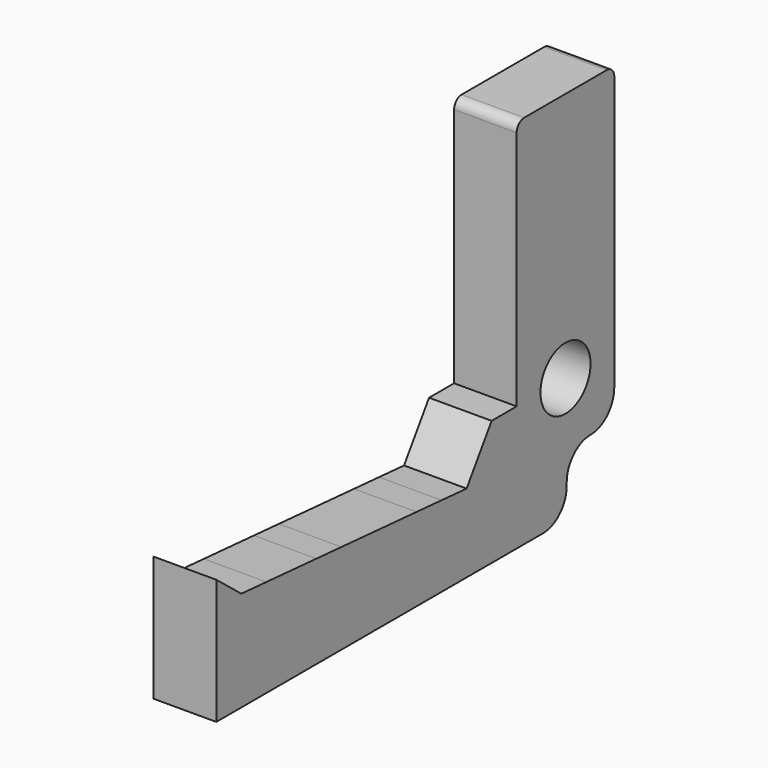
from build123d import *

# Parameters (mm, degrees)
F0_W      = 5.08
F0_H      = 9.906
F1_DEPTH  = 25.4
F2_W      = 5.08
F2_H      = 5.08
F3_DEPTH  = 5.08
F4_W      = 5.08
F4_H      = 5.08
F5_DEPTH  = 5.08
F6_DEPTH  = 5.08
F7_DEPTH  = 25.4
F9_DEPTH  = 5.081
F10_R     = 2.41299
F11_R     = 2.54
F12_DEPTH = 5.081
F13_R     = 0.762


# Not quite as in the source:
# - a fillet or chamfer is up to 0.001 mm smaller than in the source, because OpenCascade refuses the exact size


with BuildPart() as f1:
    # F0 (on Top) → F1 (new body)
    with BuildSketch(Plane.XY):
        Rectangle(F0_W, F0_H)
    extrude(amount=F1_DEPTH)

    # F2 (on face) → F3 (join)
    with BuildSketch(Plane.XZ.offset(4.953)):
        with Locations((0, 2.54)):
            Rectangle(F2_W, F2_H)
    extrude(amount=F3_DEPTH)

    # F4 (on face) → F5 (join)
    with BuildSketch(Plane(origin=(0, 0, 0), x_dir=(1, 0, 0), z_dir=(0, 0, -1))):
        with Locations((0, 7.493)):
            Rectangle(F4_W, F4_H)
    extrude(amount=F5_DEPTH)

    # F6 (add): a face of the model
    f6_faces = [f1.faces().sort_by_distance(p)[0] for p in [
        (0, -4.953, -2.54),
    ]]
    extrude(f6_faces, amount=F6_DEPTH)

    # F7 (add): a face of the model
    f7_faces = [f1.faces().sort_by_distance(p)[0] for p in [
        (0, -10.033, 0),
    ]]
    extrude(f7_faces, amount=F7_DEPTH)

    # F8 (on face) → F9 (cut, through all)
    with BuildSketch(Plane.YZ.offset(2.54)):
        Polygon((-7.493, 5.08), (-10.033, 5.08), (-10.033, 1.27), align=None)
        Polygon((-10.033, 5.08), (-12.573, 5.08), (-12.573, 1.468039654), (-10.033, 1.27), align=None)
        Polygon((-12.573, 5.08), (-15.113, 5.08), (-15.113, 1.6660793079), (-12.573, 1.468039654), align=None)
        Polygon((-15.113, 5.08), (-17.653, 5.08), (-17.653, 1.8641189619), (-15.113, 1.6660793079), align=None)
        Polygon((-20.193, 5.08), (-22.733, 5.08), (-22.733, 2.2601982699), (-20.193, 2.0621586159), align=None)
        Polygon((-17.653, 5.08), (-20.193, 5.08), (-20.193, 2.0621586159), (-17.653, 1.8641189619), align=None)
        Polygon((-22.733, 5.08), (-25.273, 5.08), (-25.273, 2.4582379238), (-22.733, 2.2601982699), align=None)
        Polygon((-25.273, 5.08), (-27.813, 5.08), (-27.813, 2.6562775778), (-25.273, 2.4582379238), align=None)
        Polygon((-27.813, 5.08), (-30.353, 5.08), (-30.353, 2.8543172318), (-27.813, 2.6562775778), align=None)
        Polygon((-30.353, 5.08), (-32.893, 5.08), (-32.893, 3.0523568857), (-30.353, 2.8543172318), align=None)
        Polygon((-32.893, 5.08), (-35.433, 5.08), (-32.893, 3.0523568857), align=None)
    extrude(amount=-F9_DEPTH, mode=Mode.SUBTRACT)

    # F10 (radius 2.413 in the source; OpenCascade refuses exactly that, so slightly less here)
    f10_edges = [f1.edges().sort_by_distance(p)[0] for p in [
        (0, 0.127, -5.08),
        (0, 0.127, 0),
        (0, 4.953, 0),
    ]]
    fillet(f10_edges, radius=F10_R)

    # F11 (on face) → F12 (cut, through all)
    with BuildSketch(Plane.YZ.offset(2.54)):
        with Locations((0, 5.08)):
            Circle(F11_R)
    extrude(amount=-F12_DEPTH, mode=Mode.SUBTRACT)

    # F13
    f13_edges = [f1.edges().sort_by_distance(p)[0] for p in [
        (0, 4.953, 25.4),
        (0, -4.953, 25.4),
    ]]
    fillet(f13_edges, radius=F13_R)


solid = f1.part
